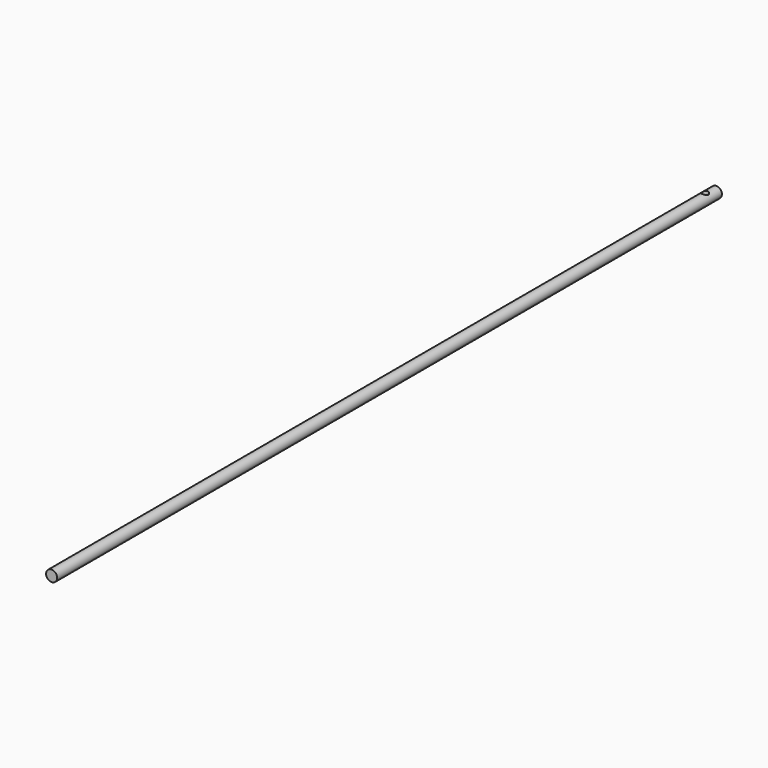
from build123d import *

# Parameters (mm, degrees)
F1_R          = 12.7094
F3_DEPTH      = 1900
F4_DEPTH      = 12.7094
F4_DEPTH_BACK = 12.7094


with BuildPart() as f3:
    # F1 (on Front) → F3 (new body)
    with BuildSketch(Plane.XZ):
        Circle(F1_R)
    extrude(amount=F3_DEPTH)

    # F2 (on Top) → F4 (cut, two sides)
    with BuildSketch(Plane.XY) as f4_sk:
        with BuildLine():
            ThreePointArc((7.5, -33), (5.3033008589, -27.6966991411), (0, -25.5))
            Line((0, -25.5), (0, -33))
            Line((0, -33), (0, -40.5))
            ThreePointArc((0, -40.5), (5.3033008589, -38.3033008589), (7.5, -33))
        make_face()
        with BuildLine():
            Line((0, -33), (0, -25.5))
            ThreePointArc((0, -25.5), (-7.5, -33), (0, -40.5))
            Line((0, -40.5), (0, -33))
        make_face()
    extrude(amount=-F4_DEPTH, mode=Mode.SUBTRACT)
    extrude(f4_sk.sketch, amount=F4_DEPTH_BACK, mode=Mode.SUBTRACT)


solid = f3.part
